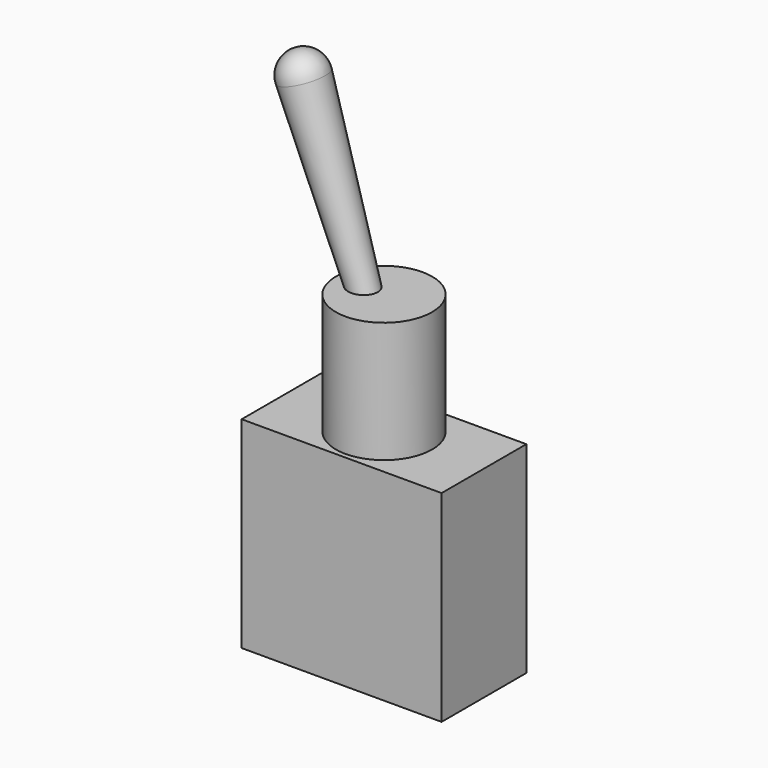
from build123d import *

# Parameters (mm, degrees)
F0_W     = 13.1826
F0_H     = 6.985
F1_DEPTH = 13.2842
F2_R     = 3.175
F3_DEPTH = 7.9756


with BuildPart() as f1:
    # F0 (on Top) → F1 (new body)
    with BuildSketch(Plane.XY):
        Rectangle(F0_W, F0_H)
    extrude(amount=F1_DEPTH)

    # F2 (on face) → F3 (join)
    with BuildSketch(Plane.XY.offset(13.2842)):
        Circle(F2_R)
    extrude(amount=F3_DEPTH)

    # F5 (on offset) → F6 (revolve)
    with BuildSketch(Plane.XZ):
        with BuildLine():
            Line((-5.8194979442, 33.6655315498), (-1.3858759776, 21.2598))
            Line((-1.3858759776, 21.2598), (-0.4049631825, 21.2598))
            Line((-0.4049631825, 21.2598), (-3.8814046251, 32.6904004058))
            ThreePointArc((-3.8814046251, 32.6904004058), (-4.6416068333, 33.5930486447), (-5.8194979442, 33.6655315498))
        make_face()
    revolve(axis=Axis((-3.6026869609, 0, 27.4626657749), (0.3365385867, 0, -0.9416696765)))


solid = f1.part
